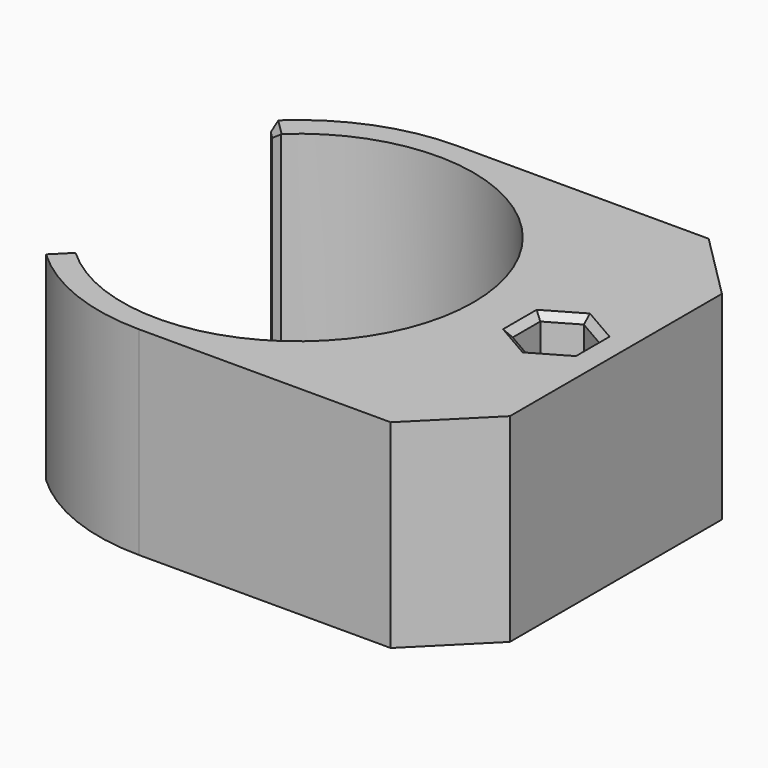
from build123d import *

# Parameters (mm, degrees)
F1_DEPTH    = 15
F2_T1_DEPTH = 17.6582428067
F2_T3_DEPTH = 17.5274686085
F2_T5_DEPTH = 4.321682988
F2_T7_DEPTH = 4.321682988
F3_SIZE     = 5
F4_SIZE     = 0.5


# Not quite as in the source:
# - a fillet or chamfer that OpenCascade refuses, or shapes differently, is made with other operations: its cross-section is extruded or revolved along the edge and cut away or added


with BuildPart() as f1:
    # F0 (on Top) → F1 (new body)
    with BuildSketch(Plane.XY):
        with BuildLine():
            ThreePointArc((0, -15), (10.6066017178, -10.6066017178), (15, 0))
            ThreePointArc((15, 0), (10.6066017178, 10.6066017178), (0, 15))
            ThreePointArc((0, 15), (-5.7402514855, 13.8581929877), (-10.6066017178, 10.6066017178))
            Line((-10.6066017178, 10.6066017178), (-9.3691648507, 9.3691648507))
            ThreePointArc((-9.3691648507, 9.3691648507), (5.0705554788, 12.2414038058), (13.25, 0))
            ThreePointArc((13.25, 0), (5.0705554788, -12.2414038058), (-9.3691648507, -9.3691648507))
            Line((-9.3691648507, -9.3691648507), (-10.6066017178, -10.6066017178))
            ThreePointArc((-10.6066017178, -10.6066017178), (-5.7402514855, -13.8581929877), (0, -15))
        make_face()
        with BuildLine():
            ThreePointArc((0, 15), (10.6066017178, 10.6066017178), (15, 0))
            ThreePointArc((15, 0), (10.6066017178, -10.6066017178), (0, -15))
            Line((0, -15), (24, -15))
            Line((24, -15), (24, 15))
            Line((24, 15), (0, 15))
        make_face()
        Polygon((19.5, -2.5980762114), (17.25, -1.2990381057), (17.25, 1.2990381057), (19.5, 2.5980762114), (21.75, 1.2990381057), (21.75, -1.2990381057), align=None, mode=Mode.SUBTRACT)
    extrude(amount=F1_DEPTH)

    # F2: chamfer of 0.5 on 8 edges, made by hand

    # F2_s2 → F2_t1 (cut)
    with BuildSketch(Plane.XY.offset(-1.3291214034)):
        with BuildLine():
            Line((-10.234549009, 10.9660387826), (-10.246950766, 10.246950766))
            Line((-10.246950766, 10.246950766), (-10.6066017178, 10.6066017178))
            ThreePointArc((-10.6066017178, 10.6066017178), (-10.4170400144, 10.7928345368), (-10.234549009, 10.9660387826))
        make_face()
        with BuildLine():
            Line((-10.246950766, -10.246950766), (-10.234549009, -10.9660387826))
            ThreePointArc((-10.234549009, -10.9660387826), (-10.4170400144, -10.7928345368), (-10.6066017178, -10.6066017178))
            Line((-10.6066017178, -10.6066017178), (-10.246950766, -10.246950766))
        make_face()
    extrude(amount=F2_T1_DEPTH, mode=Mode.SUBTRACT)

    # F2_s4 → F2_t3 (cut)
    with BuildSketch(Plane.XY.offset(-1.2637343043)):
        with BuildLine():
            Line((-9.7162878714, 9.7162878714), (-9.0222714088, 9.7036652161))
            ThreePointArc((-9.0222714088, 9.7036652161), (-9.1921439944, 9.5429025346), (-9.3691648507, 9.3691648507))
            Line((-9.3691648507, 9.3691648507), (-9.7162878714, 9.7162878714))
        make_face()
        with BuildLine():
            Line((-9.7162878714, -9.7162878714), (-9.0222714088, -9.7036652161))
            ThreePointArc((-9.0222714088, -9.7036652161), (-9.1921439944, -9.5429025346), (-9.3691648507, -9.3691648507))
            Line((-9.3691648507, -9.3691648507), (-9.7162878714, -9.7162878714))
        make_face()
    extrude(amount=F2_T3_DEPTH, mode=Mode.SUBTRACT)

    # F2_s6 → F2_t5 (cut)
    with BuildSketch(Plane(origin=(-11.5158289577, 11.5158289577, 0), x_dir=(0, 0, 1), z_dir=(0.7071067812, -0.7071067812, 0))):
        Polygon((0.5, 0), (0, -0.5), (0, 0), align=None)
        Polygon((14.5, 0), (15, -0.5), (15, 0), align=None)
    extrude(amount=F2_T5_DEPTH, mode=Mode.SUBTRACT)

    # F2_s8 → F2_t7 (cut)
    with BuildSketch(Plane(origin=(-8.4599376108, -8.4599376108, 0), x_dir=(0, 0, 1), z_dir=(-0.7071067812, -0.7071067812, 0))):
        Polygon((0.5, 0), (0, -0.5), (0, 0), align=None)
        Polygon((14.5, 0), (15, -0.5), (15, 0), align=None)
    extrude(amount=F2_T7_DEPTH, mode=Mode.SUBTRACT)

    # F3
    f3_edges = [f1.edges().sort_by_distance(p)[0] for p in [
        (24, -15, 7.5),
        (24, 15, 7.5),
    ]]
    chamfer(f3_edges, length=F3_SIZE)

    # F4
    f4_edges = [f1.edges().sort_by_distance(p)[0] for p in [
        (18.375, 1.948557, 15),
        (20.625, 1.948557, 15),
        (21.75, 0, 15),
        (20.625, -1.948557, 15),
        (18.375, -1.948557, 15),
        (17.25, 0, 15),
        (20.625, 1.948557, 0),
        (21.75, 0, 0),
        (20.625, -1.948557, 0),
        (18.375, -1.948557, 0),
        (17.25, 0, 0),
        (18.375, 1.948557, 0),
    ]]
    chamfer(f4_edges, length=F4_SIZE)


solid = f1.part
